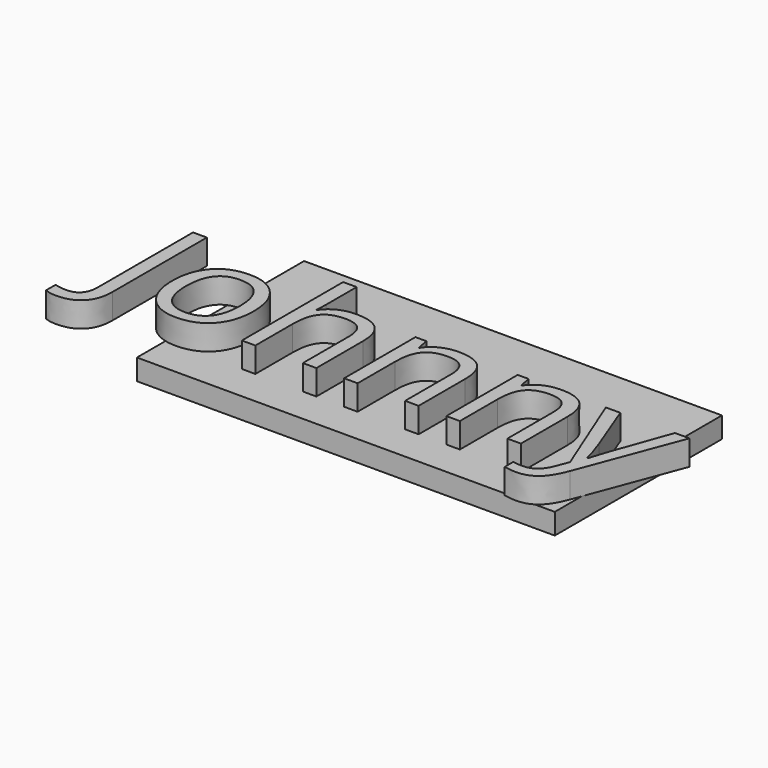
from build123d import *

# Parameters (mm, degrees)
F0_W         = 100
F0_H         = 50
F1_DEPTH     = 5
F2_DEPTH     = 5
F3_TEXT_SIZE = 39.8729630332
F4_DEPTH     = 6


# Not quite as in the source:
# - Text() gives the source's letters only with a copy of the font that has no kerning and outlines rounded to 1/6400 em; it was checked with that copy


with BuildPart() as f1:
    # F0 (on Top) → F1 (new body)
    with BuildSketch(Plane.XY):
        with Locations((25.4625026137, -7.6989527835)):
            Rectangle(F0_W, F0_H)
    extrude(amount=F1_DEPTH)

    # F0 (on Top) → F2 (join)
    with BuildSketch(Plane.XY):
        with Locations((25.4625026137, -7.6989527835)):
            Rectangle(F0_W, F0_H)
    extrude(amount=F2_DEPTH)

    # F3 (on face) → F4 (join)
    with BuildSketch(Plane.XY.offset(5)):
        with Locations((-44.4812569767, -24.0797661245)):
            Text('Johnny', F3_TEXT_SIZE, font='Open Sans', text_align=(TextAlign.LEFT, TextAlign.BOTTOM))
    extrude(amount=F4_DEPTH)


solid = f1.part
